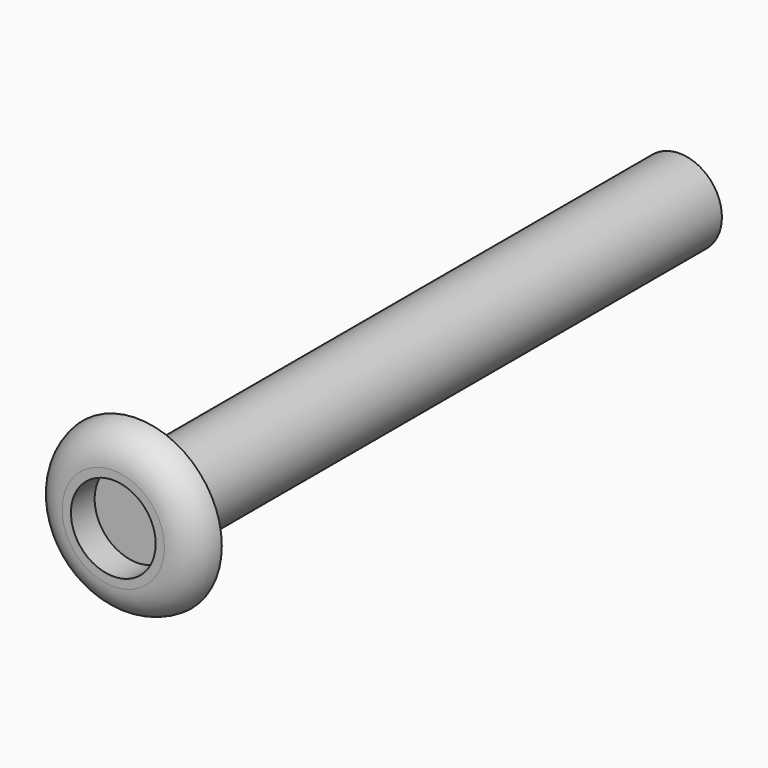
from build123d import *

# Parameters (mm, degrees)
F0_R     = 12.7
F0_R_2   = 6.35
F1_DEPTH = 4.4436082244
F3_R     = 6.35
F4_DEPTH = 101.6


# Not quite as in the source:
# - a fillet or chamfer that OpenCascade refuses, or shapes differently, is made with other operations: its cross-section is extruded or revolved along the edge and cut away or added


with BuildPart() as f1:
    # F0 (on Front) → F1 (new body)
    with BuildSketch(Plane.XZ):
        Circle(F0_R)
        Circle(F0_R_2, mode=Mode.SUBTRACT)
    extrude(amount=F1_DEPTH)

    # F2: fillet of radius 5.08 on 1 edges, made by hand

    # F2_s1 → F2_t2 (revolve, cut)
    with BuildSketch(Plane.XY):
        with BuildLine():
            ThreePointArc((12.7, 0), (11.019597377, -3.1740721214), (7.6600192949, -4.4436082244))
            Line((7.6600192949, -4.4436082244), (12.7, -4.4436082244))
            Line((12.7, -4.4436082244), (12.7, 0))
        make_face()
    revolve(axis=Axis((0, -4.4436082244, 0), (0, -1, 0)), mode=Mode.SUBTRACT)


with BuildPart() as f4:
    # F3 (on Front) → F4 (new body)
    with BuildSketch(Plane.XZ):
        Circle(F3_R)
    extrude(amount=-F4_DEPTH)


solid = Compound([f1.part, f4.part])
